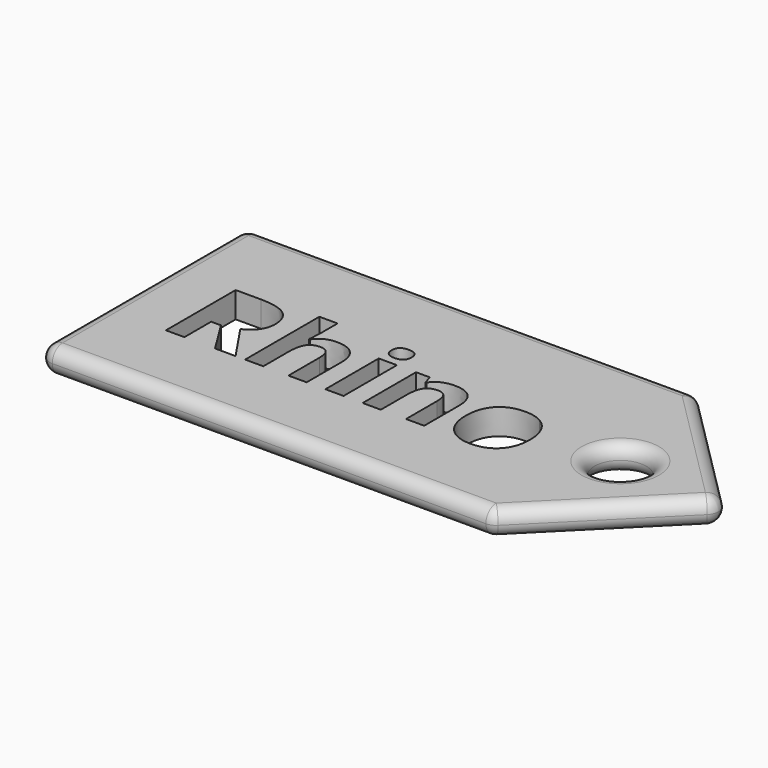
from build123d import *

# Parameters (mm, degrees)
F0_W        = 1.4087599234
F0_H        = 5.1649603066
F1_DEPTH    = 2
F2_R        = 0.99999
F3_T1_DEPTH = 2
F3_T4_ANGLE = 90
F3_T6_ANGLE = 90
F4_R        = 0.99999


# Not quite as in the source:
# - a fillet or chamfer that OpenCascade refuses, or shapes differently, is made with other operations: its cross-section is extruded or revolved along the edge and cut away or added
# - a fillet or chamfer is up to 0.001 mm smaller than in the source, because OpenCascade refuses the exact size


with BuildPart() as f1:
    # F0 (on Top) → F1 (new body)
    with BuildSketch(Plane.XY):
        Polygon((17.5, 20), (-17.5, 20), (-17.5, 0), (17.5, 0), (17.5, 10), align=None)
        with BuildLine():
            Line((-10.4563098823, 8.7796331782), (-11.217601971, 8.7796331782))
            Line((-11.217601971, 8.7796331782), (-11.217601971, 6.1882836025))
            Line((-11.217601971, 6.1882836025), (-12.6500136874, 6.1882836025))
            Line((-12.6500136874, 6.1882836025), (-12.6500136874, 12.9423487544))
            Line((-12.6500136874, 12.9423487544), (-10.6824801533, 12.9423487544))
            add(Edge.make_bspline(
                [(-10.6824801533, 12.9423487544), (-9.3047632083, 12.9423487544), (-8.6447303586, 12.4412263893)],
                knots=[0, 0, 0, 1, 1, 1], degree=2))
            add(Edge.make_bspline(
                [(-8.6447303586, 12.4412263893), (-7.9846975089, 11.9401040241), (-7.9846975089, 10.9186422119)],
                knots=[0, 0, 0, 1, 1, 1], degree=2))
            add(Edge.make_bspline(
                [(-7.9846975089, 10.9186422119), (-7.9846975089, 10.3229126745), (-8.3121270189, 9.858746236)],
                knots=[0, 0, 0, 1, 1, 1], degree=2))
            add(Edge.make_bspline(
                [(-8.3121270189, 9.858746236), (-8.6395565289, 9.3945797974), (-9.2411990145, 9.1314535998)],
                knots=[0, 0, 0, 1, 1, 1], degree=2))
            add(Edge.make_bspline(
                [(-9.2411990145, 9.1314535998), (-7.715658363, 6.853490282), (-7.2544483986, 6.1882836025)],
                knots=[0, 0, 0, 1, 1, 1], degree=2))
            Line((-7.2544483986, 6.1882836025), (-8.8435532439, 6.1882836025))
            Line((-8.8435532439, 6.1882836025), (-10.4563098823, 8.7796331782))
        make_face(mode=Mode.SUBTRACT)
        with BuildLine():
            Line((-1.7480153299, 9.5557076376), (-1.7480153299, 6.1882836025))
            Line((-1.7480153299, 6.1882836025), (-3.1567752532, 6.1882836025))
            Line((-3.1567752532, 6.1882836025), (-3.1567752532, 9.2053654531))
            add(Edge.make_bspline(
                [(-3.1567752532, 9.2053654531), (-3.1567752532, 10.3229126745), (-3.9890227211, 10.3229126745)],
                knots=[0, 0, 0, 1, 1, 1], degree=2))
            add(Edge.make_bspline(
                [(-3.9890227211, 10.3229126745), (-4.5803175472, 10.3229126745), (-4.8434437449, 9.9208321927)],
                knots=[0, 0, 0, 1, 1, 1], degree=2))
            add(Edge.make_bspline(
                [(-4.8434437449, 9.9208321927), (-5.1065699425, 9.5187517109), (-5.1065699425, 8.6185053381)],
                knots=[0, 0, 0, 1, 1, 1], degree=2))
            Line((-5.1065699425, 8.6185053381), (-5.1065699425, 6.1882836025))
            Line((-5.1065699425, 6.1882836025), (-6.5153298659, 6.1882836025))
            Line((-6.5153298659, 6.1882836025), (-6.5153298659, 13.3769504517))
            Line((-6.5153298659, 13.3769504517), (-5.1065699425, 13.3769504517))
            Line((-5.1065699425, 13.3769504517), (-5.1065699425, 11.9120175198))
            add(Edge.make_bspline(
                [(-5.1065699425, 11.9120175198), (-5.1065699425, 11.7405420203), (-5.139091158, 11.1078565563)],
                knots=[0, 0, 0, 1, 1, 1], degree=2))
            Line((-5.139091158, 11.1078565563), (-5.1716123734, 10.6924719409))
            Line((-5.1716123734, 10.6924719409), (-5.0977005201, 10.6924719409))
            add(Edge.make_bspline(
                [(-5.0977005201, 10.6924719409), (-4.6261428962, 11.4493293184), (-3.6002463728, 11.4493293184)],
                knots=[0, 0, 0, 1, 1, 1], degree=2))
            add(Edge.make_bspline(
                [(-3.6002463728, 11.4493293184), (-2.6896523405, 11.4493293184), (-2.2188338352, 10.9600328497)],
                knots=[0, 0, 0, 1, 1, 1], degree=2))
            add(Edge.make_bspline(
                [(-2.2188338352, 10.9600328497), (-1.7480153299, 10.4707363811), (-1.7480153299, 9.5557076376)],
                knots=[0, 0, 0, 1, 1, 1], degree=2))
        make_face(mode=Mode.SUBTRACT)
        with Locations((0.406515193, 8.7707637558)):
            Rectangle(F0_W, F0_H, mode=Mode.SUBTRACT)
        with BuildLine():
            Line((7.3564467561, 9.5557076376), (7.3564467561, 6.1882836025))
            Line((7.3564467561, 6.1882836025), (5.9476868327, 6.1882836025))
            Line((5.9476868327, 6.1882836025), (5.9476868327, 9.2053654531))
            add(Edge.make_bspline(
                [(5.9476868327, 9.2053654531), (5.9476868327, 9.7641390638), (5.7488639474, 10.0435258691)],
                knots=[0, 0, 0, 1, 1, 1], degree=2))
            add(Edge.make_bspline(
                [(5.7488639474, 10.0435258691), (5.5500410621, 10.3229126745), (5.1154393649, 10.3229126745)],
                knots=[0, 0, 0, 1, 1, 1], degree=2))
            add(Edge.make_bspline(
                [(5.1154393649, 10.3229126745), (4.5241445387, 10.3229126745), (4.2610183411, 9.928223378)],
                knots=[0, 0, 0, 1, 1, 1], degree=2))
            add(Edge.make_bspline(
                [(4.2610183411, 9.928223378), (3.9978921434, 9.5335340816), (3.9978921434, 8.6185053381)],
                knots=[0, 0, 0, 1, 1, 1], degree=2))
            Line((3.9978921434, 8.6185053381), (3.9978921434, 6.1882836025))
            Line((3.9978921434, 6.1882836025), (2.5891322201, 6.1882836025))
            Line((2.5891322201, 6.1882836025), (2.5891322201, 11.3532439091))
            Line((2.5891322201, 11.3532439091), (3.6652888037, 11.3532439091))
            Line((3.6652888037, 11.3532439091), (3.8545031481, 10.6924719409))
            Line((3.8545031481, 10.6924719409), (3.9328497126, 10.6924719409))
            add(Edge.make_bspline(
                [(3.9328497126, 10.6924719409), (4.169367643, 11.0664659184), (4.5825349028, 11.2578976184)],
                knots=[0, 0, 0, 1, 1, 1], degree=2))
            add(Edge.make_bspline(
                [(4.5825349028, 11.2578976184), (4.9957021626, 11.4493293184), (5.5219545579, 11.4493293184)],
                knots=[0, 0, 0, 1, 1, 1], degree=2))
            add(Edge.make_bspline(
                [(5.5219545579, 11.4493293184), (6.4236791678, 11.4493293184), (6.8900629619, 10.9622502053)],
                knots=[0, 0, 0, 1, 1, 1], degree=2))
            add(Edge.make_bspline(
                [(6.8900629619, 10.9622502053), (7.3564467561, 10.4751710923), (7.3564467561, 9.5557076376)],
                knots=[0, 0, 0, 1, 1, 1], degree=2))
        make_face(mode=Mode.SUBTRACT)
        with BuildLine():
            add(Edge.make_bspline(
                [(13.1954831645, 10.1980016425), (13.5, 9.5926635642), (13.5, 8.7796331782)],
                knots=[0, 0, 0, 1, 1, 1], degree=2))
            add(Edge.make_bspline(
                [(13.5, 8.7796331782), (13.5, 7.5186969614), (12.8347933206, 6.8069258144)],
                knots=[0, 0, 0, 1, 1, 1], degree=2))
            add(Edge.make_bspline(
                [(12.8347933206, 6.8069258144), (12.1695866411, 6.0951546674), (10.9825622776, 6.0951546674)],
                knots=[0, 0, 0, 1, 1, 1], degree=2))
            add(Edge.make_bspline(
                [(10.9825622776, 6.0951546674), (10.2390090337, 6.0951546674), (9.670626882, 6.4211059403)],
                knots=[0, 0, 0, 1, 1, 1], degree=2))
            add(Edge.make_bspline(
                [(9.670626882, 6.4211059403), (9.1022447304, 6.7470572132), (8.7977278949, 7.3568300027)],
                knots=[0, 0, 0, 1, 1, 1], degree=2))
            add(Edge.make_bspline(
                [(8.7977278949, 7.3568300027), (8.4932110594, 7.9666027922), (8.4932110594, 8.7796331782)],
                knots=[0, 0, 0, 1, 1, 1], degree=2))
            add(Edge.make_bspline(
                [(8.4932110594, 8.7796331782), (8.4932110594, 10.0450041062), (9.1532439091, 10.7471667123)],
                knots=[0, 0, 0, 1, 1, 1], degree=2))
            add(Edge.make_bspline(
                [(9.1532439091, 10.7471667123), (9.8132767588, 11.4493293184), (11.0106487818, 11.4493293184)],
                knots=[0, 0, 0, 1, 1, 1], degree=2))
            add(Edge.make_bspline(
                [(11.0106487818, 11.4493293184), (11.7542020257, 11.4493293184), (12.3225841774, 11.1263345196)],
                knots=[0, 0, 0, 1, 1, 1], degree=2))
            add(Edge.make_bspline(
                [(12.3225841774, 11.1263345196), (12.890966329, 10.8033397208), (13.1954831645, 10.1980016425)],
                knots=[0, 0, 0, 1, 1, 1], degree=2))
        make_face(mode=Mode.SUBTRACT)
        with BuildLine():
            add(Edge.make_bspline(
                [(0.4087325486, 11.9947987955), (-0.3584724884, 11.9947987955), (-0.3584724884, 12.6880919792)],
                knots=[0, 0, 0, 1, 1, 1], degree=2))
            add(Edge.make_bspline(
                [(-0.3584724884, 12.6880919792), (-0.3584724884, 13.3769504517), (0.4087325486, 13.3769504517)],
                knots=[0, 0, 0, 1, 1, 1], degree=2))
            add(Edge.make_bspline(
                [(0.4087325486, 13.3769504517), (1.1759375855, 13.3769504517), (1.1759375855, 12.6880919792)],
                knots=[0, 0, 0, 1, 1, 1], degree=2))
            add(Edge.make_bspline(
                [(1.1759375855, 12.6880919792), (1.1759375855, 12.3599233507), (0.9845058856, 12.1773610731)],
                knots=[0, 0, 0, 1, 1, 1], degree=2))
            add(Edge.make_bspline(
                [(0.9845058856, 12.1773610731), (0.7930741856, 11.9947987955), (0.4087325486, 11.9947987955)],
                knots=[0, 0, 0, 1, 1, 1], degree=2))
        make_face(mode=Mode.SUBTRACT)
        Polygon((27.5, 10), (17.5, 20), (17.5, 10), (17.5, 0), align=None)
        with BuildLine():
            ThreePointArc((21.5, 10), (19.5, 8), (17.5, 10))
            ThreePointArc((17.5, 10), (19.5, 12), (21.5, 10))
        make_face(mode=Mode.SUBTRACT)
    extrude(amount=F1_DEPTH)

    # F2 (radius 1 in the source; OpenCascade refuses exactly that, so slightly less here)
    f2_edges = [f1.edges().sort_by_distance(p)[0] for p in [
        (0, 20, 2),
        (22.5, 15, 2),
        (22.5, 5, 2),
        (22.5, 5, 0),
        (22.5, 15, 0),
        (0, 0, 2),
        (0, 0, 0),
        (17.5, 0, 1),
        (-17.5, 0, 1),
        (-17.5, 10, 2),
        (-17.5, 10, 0),
        (-17.5, 20, 1),
        (0, 20, 0),
        (17.5, 20, 1),
    ]]
    fillet(f2_edges, radius=F2_R)

    # F3: fillet of radius 1 on 2 edges, made by hand

    # F3_s2 → F3_t1 (cut)
    with BuildSketch(Plane.XY):
        with BuildLine():
            ThreePointArc((26.7928932188, 10.7071067812), (27.0857864376, 10), (26.7928932188, 9.2928932188))
            Line((26.7928932188, 9.2928932188), (27.5, 10))
            Line((27.5, 10), (26.7928932188, 10.7071067812))
        make_face()
    extrude(amount=F3_T1_DEPTH, mode=Mode.SUBTRACT)

    # F3_s3 → F3_t4 (revolve, cut)
    with BuildSketch(Plane(origin=(8.0428932188, -8.0428932188, 0), x_dir=(0, 0, 1), z_dir=(-0.7071067812, 0.7071067812, 0))):
        with BuildLine():
            ThreePointArc((0, 25.5165142945), (0.2928902899, 26.2236140046), (0.99999, 26.5165042945))
            Line((0.99999, 26.5165042945), (0, 26.5165042945))
            Line((0, 26.5165042945), (0, 25.5165142945))
        make_face()
    revolve(axis=Axis((26.0857864376, 10, 0), (0, 0, -1)), revolution_arc=F3_T4_ANGLE, mode=Mode.SUBTRACT)

    # F3_s5 → F3_t6 (revolve, cut)
    with BuildSketch(Plane(origin=(18.0428932188, 18.0428932188, 0), x_dir=(0, 0, 1), z_dir=(-0.7071067812, -0.7071067812, 0))):
        with BuildLine():
            ThreePointArc((2, -11.3743786708), (1.7071097101, -12.0814783809), (1.00001, -12.3743686708))
            Line((1.00001, -12.3743686708), (2, -12.3743686708))
            Line((2, -12.3743686708), (2, -11.3743786708))
        make_face()
    revolve(axis=Axis((26.0857864376, 10, 2), (0, 0, 1)), revolution_arc=F3_T6_ANGLE, mode=Mode.SUBTRACT)

    # F4 (radius 1 in the source; OpenCascade refuses exactly that, so slightly less here)
    f4_edges = [f1.edges().sort_by_distance(p)[0] for p in [
        (21.5, 10, 2),
        (21.5, 10, 0),
    ]]
    fillet(f4_edges, radius=F4_R)


solid = f1.part
